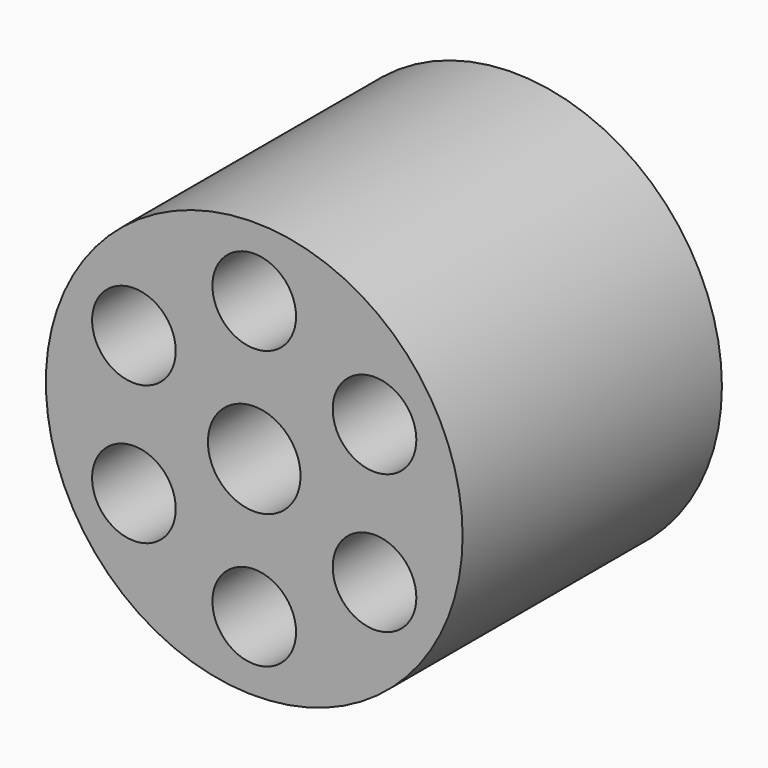
from build123d import *

# Parameters (mm, degrees)
F0_R            = 22.5
F0_R_2          = 4.515
F0_R_3          = 5
F1_DEPTH        = 17.5
F2_R            = 4.825
F3_DEPTH        = 19.15
F3_COPIES_COUNT = 6


# Not quite as in the source:
# - a pattern or mirror of a feature is missing from the dataset's text; its kind, count and spacing are read off the source's solid


with BuildPart() as f1:
    # F0 (on Front) → F1 (new body, symmetric)
    with BuildSketch(Plane.XZ):
        Circle(F0_R)
        with Locations((-12.9903810568, -7.5)):
            Circle(F0_R_2, mode=Mode.SUBTRACT)
        with Locations((0, -15)):
            Circle(F0_R_2, mode=Mode.SUBTRACT)
        with Locations((12.9903810568, -7.5)):
            Circle(F0_R_2, mode=Mode.SUBTRACT)
        with Locations((-12.9903810568, 7.5)):
            Circle(F0_R_2, mode=Mode.SUBTRACT)
        Circle(F0_R_3, mode=Mode.SUBTRACT)
        with Locations((12.9903810568, 7.5)):
            Circle(F0_R_2, mode=Mode.SUBTRACT)
        with Locations((0, 15)):
            Circle(F0_R_2, mode=Mode.SUBTRACT)
    extrude(amount=F1_DEPTH, both=True)

    # F2 (on face) → F3 (cut)
    with BuildSketch(Plane(origin=(0, 17.5, 0), x_dir=(-1, 0, 0), z_dir=(0, 1, 0))):
        with Locations((0, 15)):
            Circle(F2_R)
    f3 = extrude(amount=-F3_DEPTH, mode=Mode.SUBTRACT)

    # F3_copies: F3 ×6 about axis
    f3_copies_axis = Axis((0, 0, 0), (0, 1, 0))
    for i in range(1, F3_COPIES_COUNT):
        add(f3.rotate(f3_copies_axis, i * 360 / F3_COPIES_COUNT), mode=Mode.SUBTRACT)


solid = f1.part
